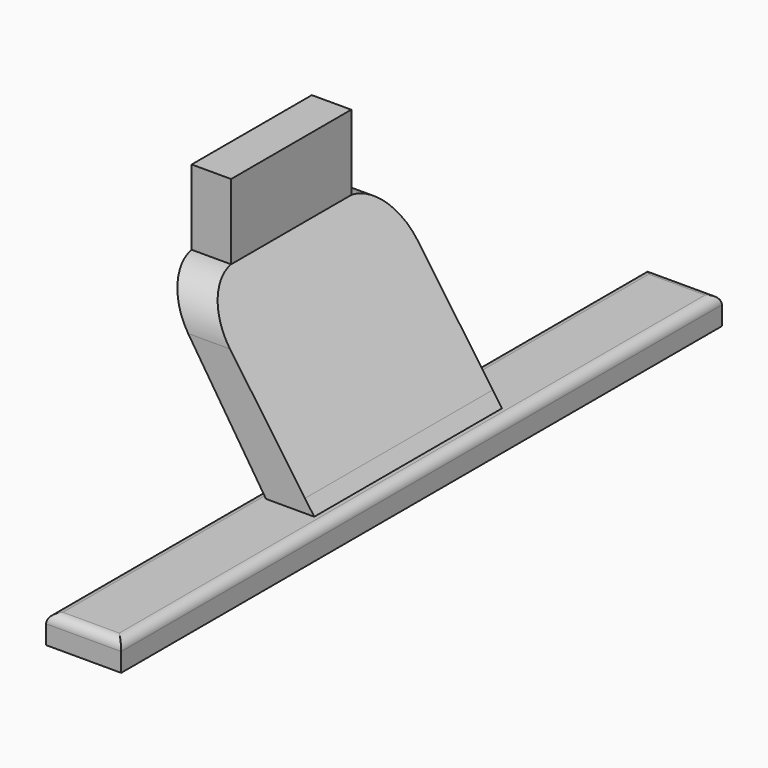
from build123d import *

# Parameters (mm, degrees)
F0_W        = 4.2
F0_H        = 16
F1_DEPTH    = 8
F4_DEPTH    = 12.5
F5_W        = 8
F5_H        = 80
F6_DEPTH    = 3
F7_R        = 1
F8_T1_DEPTH = 29.0746859277


# Not quite as in the source:
# - a fillet or chamfer that OpenCascade refuses, or shapes differently, is made with other operations: its cross-section is extruded or revolved along the edge and cut away or added


with BuildPart() as f1:
    # F0 (on Top) → F1 (new body)
    with BuildSketch(Plane.XY):
        Rectangle(F0_W, F0_H)
    extrude(amount=F1_DEPTH)

    # F3 (on face) → F4 (join, symmetric)
    with BuildSketch(Plane.XZ):
        Polygon((13.571528727, -16.3830408858), (2.1, 0), (-0.9, 0), (11.558498512, -17.792579817), align=None)
        Polygon((14.558498512, -17.792579817), (13.571528727, -16.3830408858), (11.558498512, -17.792579817), align=None)
        Polygon((11.558498512, -17.792579817), (-0.9, 0), (-2.1, 0), (9.4175692648, -17.792579817), align=None)
    extrude(amount=F4_DEPTH, both=True)

    # F5 (on face) → F6 (join)
    with BuildSketch(Plane(origin=(0, 0, -17.792579817), x_dir=(1, 0, 0), z_dir=(0, 0, -1))):
        with Locations((11.9880338884, 0)):
            Rectangle(F5_W, F5_H)
    extrude(amount=F6_DEPTH)

    # F7
    f7_edges = [f1.edges().sort_by_distance(p)[0] for p in [
        (15.988034, 0, -17.79258),
        (11.988034, 40, -17.79258),
        (7.988034, 0, -17.79258),
        (11.988034, -40, -17.79258),
    ]]
    fillet(f7_edges, radius=F7_R)

    # F8: fillet of radius 5 on 2 edges, made by hand

    # F8_s2 → F8_t1 (cut)
    with BuildSketch(Plane.YZ.offset(-14.5373429638)):
        with BuildLine():
            ThreePointArc((-12.5, -4.9749371855), (-11.2080992435, -1.6208352193), (-8, 0))
            Line((-8, 0), (-12.5, 0))
            Line((-12.5, 0), (-12.5, -4.9749371855))
        make_face()
        with BuildLine():
            ThreePointArc((12.5, -4.9749371855), (11.2080992435, -1.6208352193), (8, 0))
            Line((8, 0), (12.5, 0))
            Line((12.5, 0), (12.5, -4.9749371855))
        make_face()
    extrude(amount=F8_T1_DEPTH, mode=Mode.SUBTRACT)


solid = f1.part
